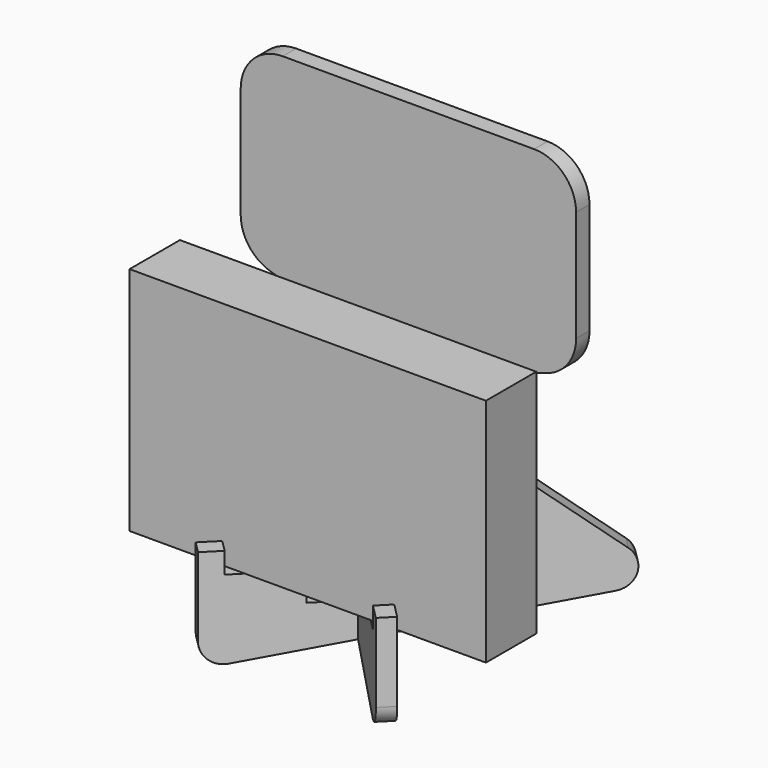
from build123d import *

# Parameters (mm, degrees)
F0_W      = 85
F0_H      = 55
F1_DEPTH  = 15
F5_DEPTH  = 4
F7_W      = 13.6952600442
F7_H      = 45
F8_DEPTH  = 25
F9_W      = 4
F9_H      = 1.4558660838
F10_DEPTH = 25
F11_W     = 4
F11_H     = 12.2237176445
F12_DEPTH = 4
F15_DEPTH = 4
F16_W     = 6.8639610307
F16_H     = 10
F17_DEPTH = 25
F18_W     = 7
F18_H     = 10
F19_DEPTH = 25
F20_R     = 10


with BuildPart() as f1:
    # F0 (on Front) → F1 (new body)
    with BuildSketch(Plane.XZ):
        Rectangle(F0_W, F0_H)
    extrude(amount=F1_DEPTH)

    # F9 (on face) → F10 (cut)
    with BuildSketch(Plane(origin=(2.8284271247, 2.8284271247, 0), x_dir=(-0.7071067812, 0.7071067812, 0), z_dir=(0.7071067812, 0.7071067812, 0))):
        with Locations((2, -49.5630876647)):
            Rectangle(F9_W, F9_H)
    extrude(amount=-F10_DEPTH, mode=Mode.SUBTRACT)


with BuildPart() as f5:
    # F4 (on line) → F5 (new body)
    with BuildSketch(Plane(origin=(0, 0, 0), x_dir=(-0.7071067812, -0.7071067812, 0), z_dir=(-0.7071067812, 0.7071067812, 0))):
        with BuildLine():
            Line((25, -27.5), (0, -27.5))
            Line((0, -27.5), (0, 3.7089792934))
            ThreePointArc((0, 3.7089792934), (-2.8284017695, 8.2127733746), (-8.1136644502, 7.6211517963))
            Line((-8.1136644502, 7.6211517963), (-50.6545456419, -26.236769691))
            ThreePointArc((-50.6545456419, -26.236769691), (-52.3730201924, -31.4336338606), (-48.3005526751, -35.0908951718))
            Line((-48.3005526751, -35.0908951718), (24.2403285166, -46.2417982796))
            ThreePointArc((24.2403285166, -46.2417982796), (28.2558902456, -45.0944702776), (30, -41.2998453016))
            Line((30, -41.2998453016), (30, -22.5))
            Line((30, -22.5), (25, -22.5))
            Line((25, -22.5), (25, -27.5))
        make_face()
    extrude(amount=F5_DEPTH)


with BuildPart() as f6_1:
    # F6: instance of F5
    add(f5.part.mirror(Plane.YZ))

    # F11 (on face) → F12 (cut)
    with BuildSketch(Plane(origin=(0, 0, 0), x_dir=(0.7071067812, -0.7071067812, 0), z_dir=(-0.7071067812, -0.7071067812, 0))):
        with Locations((-2, -40.4028795288)):
            Rectangle(F11_W, F11_H)
    extrude(amount=-F12_DEPTH, mode=Mode.SUBTRACT)

    # F16 (on face) → F17 (cut)
    with BuildSketch(Plane(origin=(0, 0, 0), x_dir=(0.7071067812, -0.7071067812, 0), z_dir=(-0.7071067812, -0.7071067812, 0))):
        with Locations((-24.6451839509, -15)):
            Rectangle(F16_W, F16_H)
    extrude(amount=-F17_DEPTH, mode=Mode.SUBTRACT)


with BuildPart() as f5_1:
    add(f5.part)

    # F7 (on face) → F8 (cut)
    with BuildSketch(Plane(origin=(0, 0, 0), x_dir=(0.7071067812, 0.7071067812, 0), z_dir=(0.7071067812, -0.7071067812, 0))):
        with Locations((-2.8476300221, -11.7910207066)):
            Rectangle(F7_W, F7_H)
    extrude(amount=-F8_DEPTH, mode=Mode.SUBTRACT)

    # F18 (on face) → F19 (cut)
    with BuildSketch(Plane(origin=(0, 0, 0), x_dir=(0.7071067812, 0.7071067812, 0), z_dir=(0.7071067812, -0.7071067812, 0))):
        with Locations((24.7132034356, -15)):
            Rectangle(F18_W, F18_H)
    extrude(amount=-F19_DEPTH, mode=Mode.SUBTRACT)


with BuildPart() as f15:
    # F14 (on offset) → F15 (new body)
    with BuildSketch(Plane.XZ.offset(-15)):
        with BuildLine():
            Line((40, 64.0720436681), (-40, 64.0720436681))
            Line((-40, 64.0720436681), (-40, 19.0720436681))
            ThreePointArc((-40, 19.0720436681), (-22.509087408, 13.4541849351), (-10, 0))
            Line((-10, 0), (-10, -10))
            Line((-10, -10), (-20, -10))
            Line((-20, -10), (-20, -20))
            Line((-20, -20), (-10, -20))
            Line((-10, -20), (10, -20))
            Line((10, -20), (20, -20))
            Line((20, -20), (20, -10))
            Line((20, -10), (10, -10))
            Line((10, -10), (10, 0))
            ThreePointArc((10, 0), (22.509087408, 13.4541849351), (40, 19.0720436681))
            Line((40, 19.0720436681), (40, 64.0720436681))
        make_face()
    extrude(amount=-F15_DEPTH)

    # F20
    f20_edges = [f15.edges().sort_by_distance(p)[0] for p in [
        (40, 17, 64.072044),
        (40, 17, 19.072044),
        (-40, 17, 64.072044),
        (-40, 17, 19.072044),
    ]]
    fillet(f20_edges, radius=F20_R)


solid = Compound([f1.part, f6_1.part, f5_1.part, f15.part])
